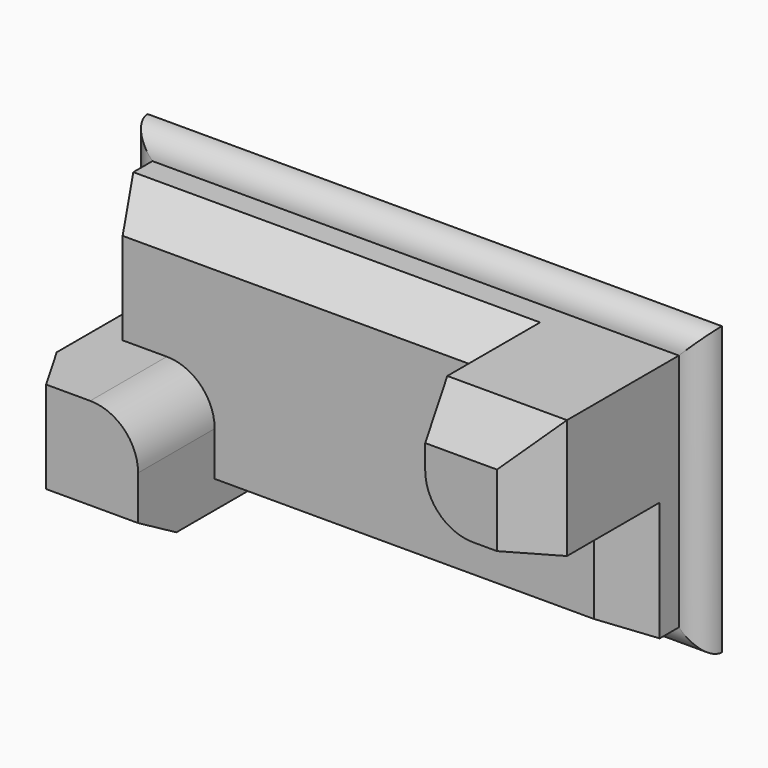
from build123d import *

# Parameters (mm, degrees)
F1_DEPTH    = 25.4
F0_W        = 152.4
F0_H        = 76.2
F2_DEPTH    = 6.35
F3_DEPTH    = 50.8
F4_R        = 6.34999
F5_C1_SIZE2 = 7.3323484187
F5_C1_SIZE  = 12.7
F5_C2_SIZE2 = 7.3323484187
F5_C2_SIZE  = 12.7
F5_C3_SIZE2 = 12.7
F5_C3_SIZE  = 7.3323484187
F5_C4_SIZE2 = 7.3323484187
F5_C4_SIZE  = 12.7
F5_C5_SIZE2 = 7.3323484187
F5_C5_SIZE  = 12.7
F5_C6_SIZE2 = 12.7
F5_C6_SIZE  = 7.3323484187
F5_C7_SIZE2 = 7.3323484187
F5_C7_SIZE  = 12.7
F5_C8_SIZE2 = 7.3323484187
F5_C8_SIZE  = 12.7


# Not quite as in the source:
# - a fillet or chamfer is up to 0.001 mm smaller than in the source, because OpenCascade refuses the exact size


with BuildPart() as f1:
    # F0 (on Front) → F1 (new body)
    with BuildSketch(Plane.XZ):
        with BuildLine():
            Line((114.3, -6.35), (6.35, -6.35))
            Line((6.35, -6.35), (6.35, -38.1))
            Line((6.35, -38.1), (25.4, -38.1))
            ThreePointArc((25.4, -38.1), (34.3802561211, -41.8197438789), (38.1, -50.8))
            Line((38.1, -50.8), (38.1, -69.85))
            Line((38.1, -69.85), (146.05, -69.85))
            Line((146.05, -69.85), (146.05, -38.1))
            Line((146.05, -38.1), (127, -38.1))
            ThreePointArc((127, -38.1), (118.0197438789, -34.3802561211), (114.3, -25.4))
            Line((114.3, -25.4), (114.3, -6.35))
        make_face()
    extrude(amount=F1_DEPTH)

    # F0 (on Front) → F2 (join)
    with BuildSketch(Plane.XZ):
        with Locations((76.2, -38.1)):
            Rectangle(F0_W, F0_H)
        Polygon((6.35, -38.1), (6.35, -6.35), (114.3, -6.35), (146.05, -6.35), (146.05, -38.1), (146.05, -69.85), (38.1, -69.85), (6.35, -69.85), align=None, mode=Mode.SUBTRACT)
    extrude(amount=F2_DEPTH)

    # F0 (on Front) → F3 (join)
    with BuildSketch(Plane.XZ):
        with BuildLine():
            Line((25.4, -38.1), (6.35, -38.1))
            Line((6.35, -38.1), (6.35, -69.85))
            Line((6.35, -69.85), (38.1, -69.85))
            Line((38.1, -69.85), (38.1, -50.8))
            ThreePointArc((38.1, -50.8), (34.3802561211, -41.8197438789), (25.4, -38.1))
        make_face()
        with BuildLine():
            Line((146.05, -6.35), (114.3, -6.35))
            Line((114.3, -6.35), (114.3, -25.4))
            ThreePointArc((114.3, -25.4), (118.0197438789, -34.3802561211), (127, -38.1))
            Line((127, -38.1), (146.05, -38.1))
            Line((146.05, -38.1), (146.05, -6.35))
        make_face()
    extrude(amount=F3_DEPTH)

    # F4 (radius 6.35 in the source; OpenCascade refuses exactly that, so slightly less here)
    f4_edges = [f1.edges().sort_by_distance(p)[0] for p in [
        (76.2, -6.35, -76.2),
        (0, -6.35, -38.1),
        (152.4, -6.35, -38.1),
        (76.2, -6.35, 0),
    ]]
    fillet(f4_edges, radius=F4_R)

    # F5: chamfer of 12.7 x 7.3323484187 on 8 edges, made by hand

    # F5_c1
    f5_c1_edges = [f1.edges().sort_by_distance(p)[0] for p in [
        (6.35, -25.4, -22.225),
    ]]
    f5_c1_side = f1.faces().sort_by_distance((6.35, -25.2533530316, -22.225))[0]
    chamfer(f5_c1_edges, length=F5_C1_SIZE, length2=F5_C1_SIZE2, reference=f5_c1_side)

    # F5_c2
    f5_c2_edges = [f1.edges().sort_by_distance(p)[0] for p in [
        (6.35, -50.8, -53.975),
    ]]
    f5_c2_side = f1.faces().sort_by_distance((6.35, -50.6533530316, -53.975))[0]
    chamfer(f5_c2_edges, length=F5_C2_SIZE, length2=F5_C2_SIZE2, reference=f5_c2_side)

    # F5_c3
    f5_c3_edges = [f1.edges().sort_by_distance(p)[0] for p in [
        (130.175, -50.8, -6.35),
    ]]
    f5_c3_side = f1.faces().sort_by_distance((130.175, -50.6533530316, -6.35))[0]
    chamfer(f5_c3_edges, length=F5_C3_SIZE, length2=F5_C3_SIZE2, reference=f5_c3_side)

    # F5_c4
    f5_c4_edges = [f1.edges().sort_by_distance(p)[0] for p in [
        (63.9911742094, -25.4, -6.35),
    ]]
    f5_c4_side = f1.faces().sort_by_distance((63.9911742094, -25.2533530316, -6.35))[0]
    chamfer(f5_c4_edges, length=F5_C4_SIZE, length2=F5_C4_SIZE2, reference=f5_c4_side)

    # F5_c5
    f5_c5_edges = [f1.edges().sort_by_distance(p)[0] for p in [
        (146.05, -25.4, -53.975),
    ]]
    f5_c5_side = f1.faces().sort_by_distance((146.05, -25.2533530316, -53.975))[0]
    chamfer(f5_c5_edges, length=F5_C5_SIZE, length2=F5_C5_SIZE2, reference=f5_c5_side)

    # F5_c6
    f5_c6_edges = [f1.edges().sort_by_distance(p)[0] for p in [
        (146.05, -50.8, -28.575),
    ]]
    f5_c6_side = f1.faces().sort_by_distance((146.05, -50.6533530316, -28.575))[0]
    chamfer(f5_c6_edges, length=F5_C6_SIZE, length2=F5_C6_SIZE2, reference=f5_c6_side)

    # F5_c7
    f5_c7_edges = [f1.edges().sort_by_distance(p)[0] for p in [
        (25.8911742094, -50.8, -69.85),
    ]]
    f5_c7_side = f1.faces().sort_by_distance((25.8911742094, -50.6533530316, -69.85))[0]
    chamfer(f5_c7_edges, length=F5_C7_SIZE, length2=F5_C7_SIZE2, reference=f5_c7_side)

    # F5_c8
    f5_c8_edges = [f1.edges().sort_by_distance(p)[0] for p in [
        (88.4088257906, -25.4, -69.85),
    ]]
    f5_c8_side = f1.faces().sort_by_distance((88.4088257906, -25.2533530316, -69.85))[0]
    chamfer(f5_c8_edges, length=F5_C8_SIZE, length2=F5_C8_SIZE2, reference=f5_c8_side)


solid = f1.part
